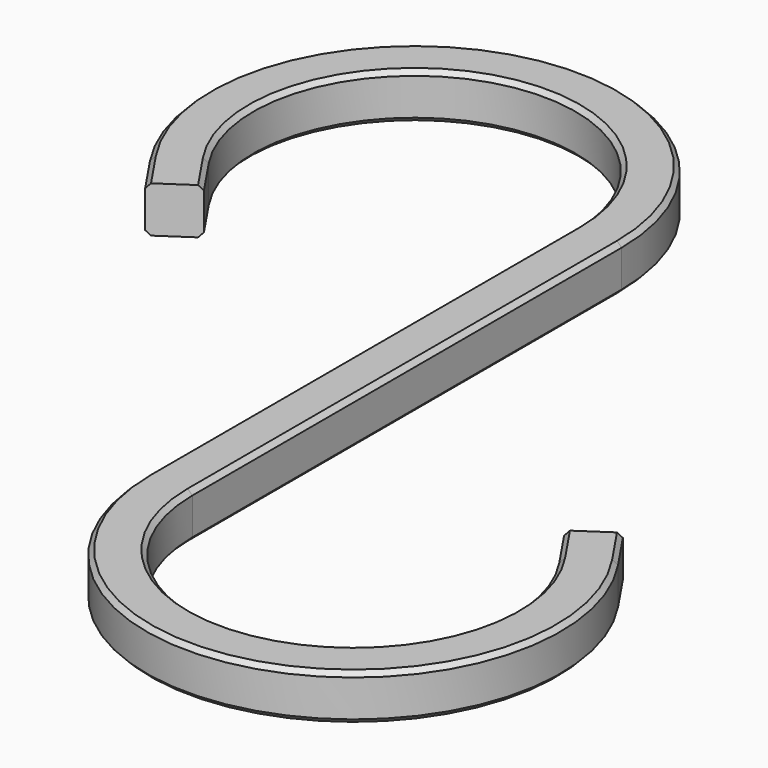
from build123d import *

# Parameters (mm, degrees)
F1_W    = 5
F1_H    = 5
F3_SIZE = 0.5


with BuildPart() as f2:
    # F2: sweep along a path in F0
    with BuildLine(Plane.XY) as f2_path:
        Line((-33.7847869337, 13.8033740678), (-36.5807514511, 17.9485619306))
        ThreePointArc((-36.5807514511, 17.9485619306), (-25.8474340945, 48.2585151193), (0, 29.13242))
        Line((0, 29.13242), (0, -29.13242))
        ThreePointArc((0, -29.13242), (25.8474340945, -48.2585151193), (36.5807514511, -17.9485619306))
        Line((36.5807514511, -17.9485619306), (33.7847869337, -13.8033740678))
    # F1 (on Front) → F2 (sweep)
    with BuildSketch(Plane.XZ):
        Rectangle(F1_W, F1_H)
    sweep(path=f2_path.line)

    # F3
    f3_edges = [f2.edges().sort_by_distance(p)[0] for p in [
        (-2.5, 0, -2.5),
        (-26.578363, 50.649277, -2.5),
        (-26.578363, 50.649277, 2.5),
        (-2.5, 0, 2.5),
    ]]
    chamfer(f3_edges, length=F3_SIZE)


solid = f2.part
